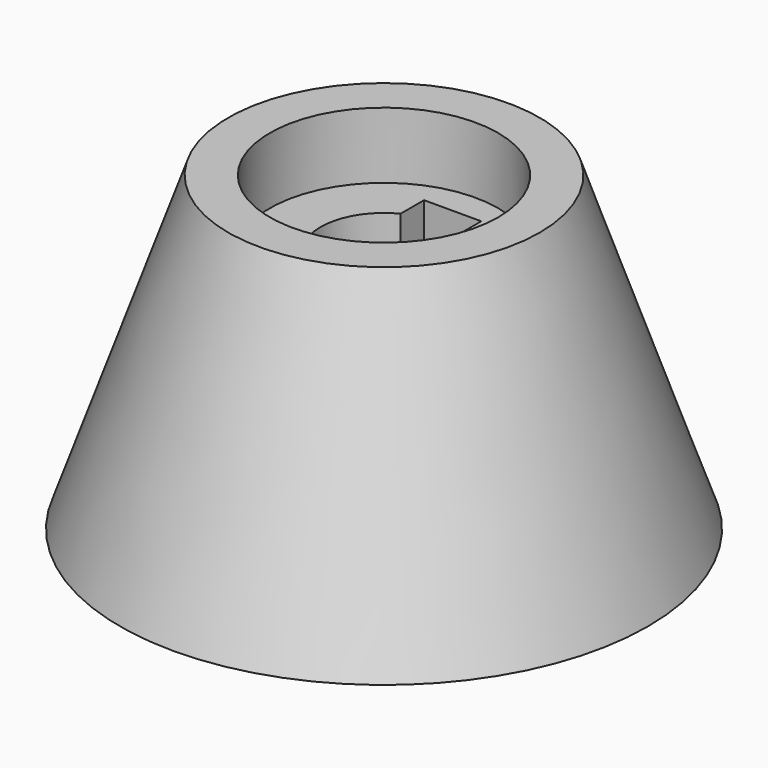
from build123d import *

# Parameters (mm, degrees)
F3_R      = 14
F4_DEPTH  = 30
F6_R      = 4.5
F7_DEPTH  = 27
F5_R      = 7.75
F8_DEPTH  = 11
F10_DEPTH = 25


# Not quite as in the source:
# - a feature names something its author has since deleted; it is built from what else it names


with BuildPart() as f2:
    # F0 (on Front) → F2 (revolve)
    with BuildSketch(Plane.XZ):
        Polygon((32.2950072587, 0), (19.05, 38.1), (13.97, 38.1), (13.97, 0), align=None)
    revolve(axis=Axis((0, 0, 18.1650817394), (0, 0, 1)))

    # F3 (on Top) → F4 (join)
    with BuildSketch(Plane.XY):
        Circle(F3_R)
    extrude(amount=F4_DEPTH)

    # F6 (on face) → F7 (cut)
    with BuildSketch(Plane.XY.offset(30)):
        Circle(F6_R)
    extrude(amount=-F7_DEPTH, mode=Mode.SUBTRACT)

    # F5 (on face) → F8 (cut)
    with BuildSketch(Plane.XY.offset(30)):
        Circle(F5_R)
    extrude(amount=-F8_DEPTH, mode=Mode.SUBTRACT)

    # F9 (on face) → F10 (cut)
    with BuildSketch(Plane.XY.offset(30)):
        Polygon((-3.5, 0), (0, 0), (3.5, 0), (3.5, 10.5), (-3.5, 10.5), align=None)
    extrude(amount=-F10_DEPTH, mode=Mode.SUBTRACT)


solid = f2.part
